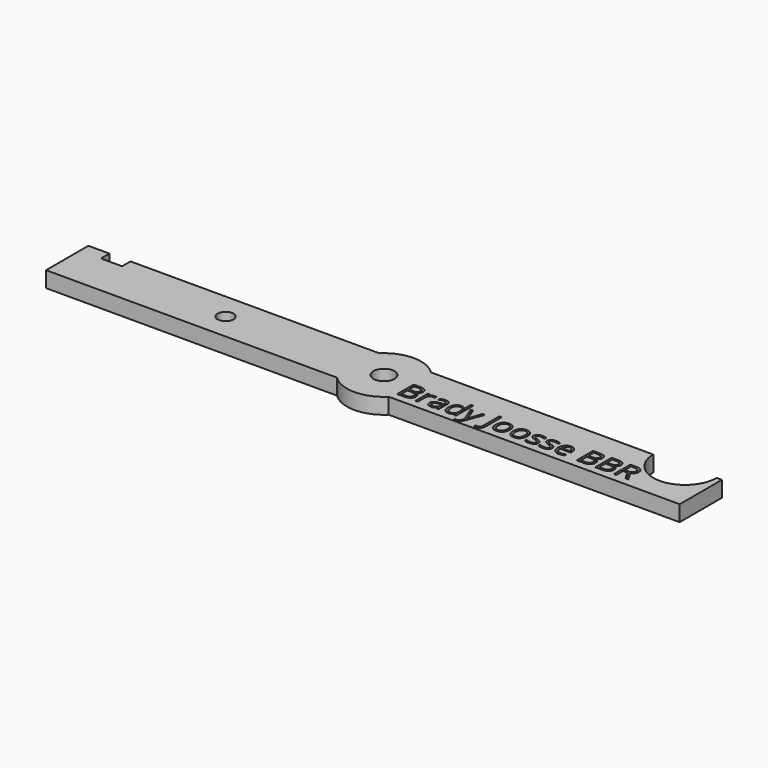
from build123d import *

# Parameters (mm, degrees)
F0_R         = 1.5
F0_R_2       = 2
F1_DEPTH     = 3
F2_TEXT_SIZE = 5.4460584781
F3_DEPTH     = 25


# Not quite as in the source:
# - Text() gives the source's letters only with a copy of the font that has no kerning and outlines rounded to 1/6400 em; it was checked with that copy


with BuildPart() as f1:
    # F0 (on Top) → F1 (new body)
    with BuildSketch(Plane.XY):
        with BuildLine():
            Line((-60, 5), (-60, -5))
            Line((-60, -5), (-4.8989794856, -5))
            ThreePointArc((-4.8989794856, -5), (-7, 0), (-4.8989794856, 5))
            Line((-4.8989794856, 5), (-52, 5))
            Line((-52, 5), (-52, 3))
            Line((-52, 3), (-56, 3))
            Line((-56, 3), (-56, 5))
            Line((-56, 5), (-60, 5))
        make_face()
        with Locations((-30, 0)):
            Circle(F0_R, mode=Mode.SUBTRACT)
        with BuildLine():
            ThreePointArc((7, 0), (6.4534043883, -2.7117470016), (4.8989794856, -5))
            Line((4.8989794856, -5), (60, -5))
            Line((60, -5), (60, 5))
            Line((60, 5), (59, 5))
            ThreePointArc((59, 5), (53, -1), (47, 5))
            Line((47, 5), (4.8989794856, 5))
            ThreePointArc((4.8989794856, 5), (6.4534043883, 2.7117470016), (7, 0))
        make_face()
        with BuildLine():
            Line((4.8989794856, -5), (-4.8989794856, -5))
            ThreePointArc((-4.8989794856, -5), (0, -7), (4.8989794856, -5))
        make_face()
        with BuildLine():
            ThreePointArc((-4.8989794856, 5), (-7, 0), (-4.8989794856, -5))
            Line((-4.8989794856, -5), (4.8989794856, -5))
            ThreePointArc((4.8989794856, -5), (6.4534043883, -2.7117470016), (7, 0))
            ThreePointArc((7, 0), (6.4534043883, 2.7117470016), (4.8989794856, 5))
            Line((4.8989794856, 5), (-4.8989794856, 5))
        make_face()
        Circle(F0_R_2, mode=Mode.SUBTRACT)
        with BuildLine():
            ThreePointArc((4.8989794856, 5), (0, 7), (-4.8989794856, 5))
            Line((-4.8989794856, 5), (4.8989794856, 5))
        make_face()
    extrude(amount=F1_DEPTH)

    # F2 (on face) → F3 (cut)
    with BuildSketch(Plane.XY.offset(3)):
        with Locations((4.8050377518, -3.547298682)):
            Text('Brady Joosse BBR', F2_TEXT_SIZE, font='Open Sans', text_align=(TextAlign.LEFT, TextAlign.BOTTOM))
    extrude(amount=-F3_DEPTH, mode=Mode.SUBTRACT)


solid = f1.part
